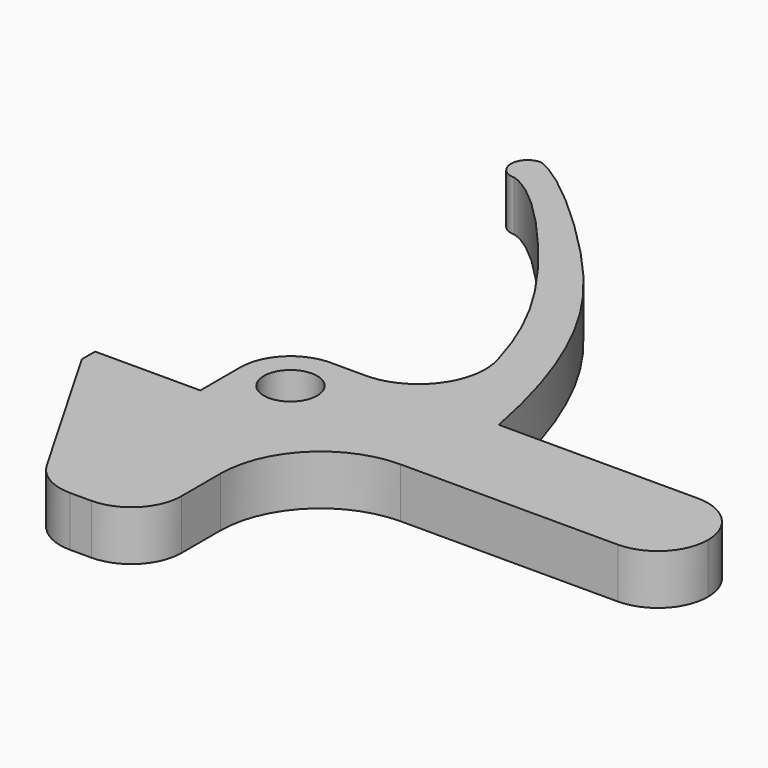
from build123d import *

# Parameters (mm, degrees)
F0_R     = 1.6
F0_W     = 6.3
F0_H     = 1
F1_DEPTH = 3
F2_R     = 2.99999
F3_R     = 6
F4_R     = 4


# Not quite as in the source:
# - a fillet or chamfer is up to 0.001 mm smaller than in the source, because OpenCascade refuses the exact size
# - a feature names something its author has since deleted; it is built from what else it names


with BuildPart() as f1:
    # F0 (on Top) → F1 (new body)
    with BuildSketch(Plane.XY):
        with BuildLine():
            ThreePointArc((0, 3), (-2.1213203436, 2.1213203436), (-3, 0))
            Line((-3, 0), (-3, -3))
            Line((-3, -3), (-3, -4))
            Line((-3, -4), (-9.3, -4))
            Line((-9.3, -4), (-3, -14.9119200877))
            Line((-3, -14.9119200877), (3, -14.9119200877))
            Line((3, -14.9119200877), (3, -3))
            Line((3, -3), (25, -3))
            Line((25, -3), (25, 3))
            Line((25, 3), (10.0770951748, 3))
            Line((10.0770951748, 3), (7.0770951748, 3))
            Line((7.0770951748, 3), (0, 3))
        make_face()
        Circle(F0_R, mode=Mode.SUBTRACT)
        with Locations((-6.15, -3.5)):
            Rectangle(F0_W, F0_H)
        with BuildLine():
            add(Edge.make_bspline(
                [(7.0770951748, 3), (6.4332614255, 6.4067024909), (5.2223697544, 11.3722601643), (1.0114116485, 17.6559878049), (-3.6425327417, 22.6266458631), (-5, 23)],
                knots=[0, 0, 0, 0, 0.3461061531, 0.6777539699, 1, 1, 1, 1], degree=3))
            Line((7.0770951748, 3), (10.0770951748, 3))
            add(Edge.make_bspline(
                [(10.0770951748, 3), (9.3764700877, 6.6524697116), (7.4550072041, 12.4304500602), (2.9271463912, 18.7046739484), (-3.554672909, 24.5379839434), (-5, 25)],
                knots=[0, 0, 0, 0, 0.3430568532, 0.6625508471, 1, 1, 1, 1], degree=3))
            ThreePointArc((-5, 25), (-6, 24), (-5, 23))
        make_face()
    extrude(amount=F1_DEPTH)

    # F2 (radius 3 in the source; OpenCascade refuses exactly that, so slightly less here)
    f2_edges = [f1.edges().sort_by_distance(p)[0] for p in [
        (-3, -14.91192, 1.5),
        (3, -14.91192, 1.5),
        (25, -3, 1.5),
        (25, 3, 1.5),
    ]]
    fillet(f2_edges, radius=F2_R)

    # F3
    f3_edges = [f1.edges().sort_by_distance(p)[0] for p in [
        (3, -3, 1.5),
    ]]
    fillet(f3_edges, radius=F3_R)

    # F4
    f4_edges = [f1.edges().sort_by_distance(p)[0] for p in [
        (7.077095, 3, 1.5),
    ]]
    fillet(f4_edges, radius=F4_R)


solid = f1.part
